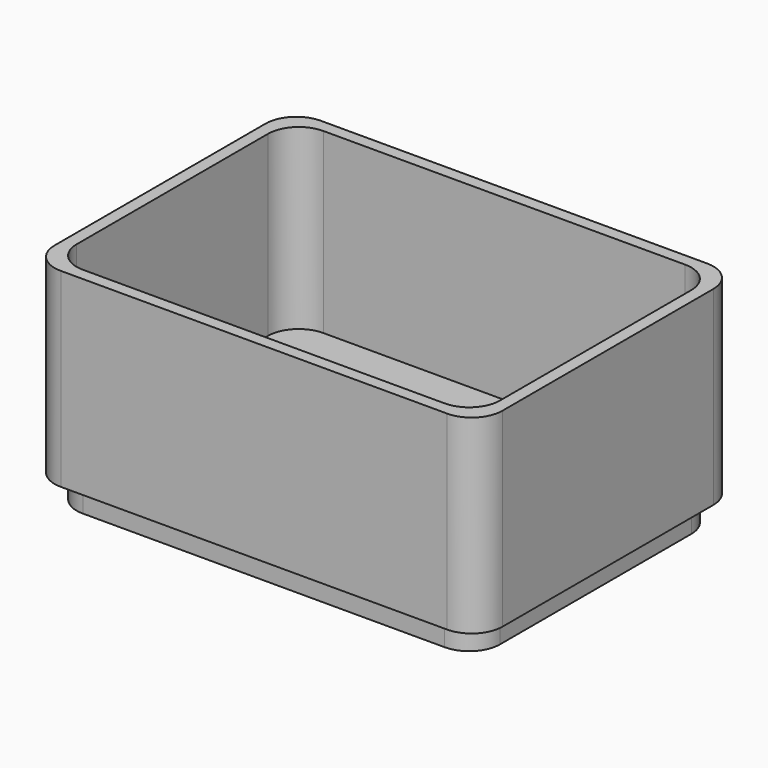
from build123d import *

# Parameters (mm, degrees)
F1_DEPTH = 6
F2_DEPTH = 35
F3_DEPTH = 4


with BuildPart() as f1:
    # F0 (on Top) → F1 (new body)
    with BuildSketch(Plane.XY):
        with BuildLine():
            Line((31.5, 26.5), (-31.5, 26.5))
            ThreePointArc((-31.5, 26.5), (-35.0355339059, 25.0355339059), (-36.5, 21.5))
            Line((-36.5, 21.5), (-36.5, -21.5))
            ThreePointArc((-36.5, -21.5), (-35.0355339059, -25.0355339059), (-31.5, -26.5))
            Line((-31.5, -26.5), (31.5, -26.5))
            ThreePointArc((31.5, -26.5), (35.0355339059, -25.0355339059), (36.5, -21.5))
            Line((36.5, -21.5), (36.5, 21.5))
            ThreePointArc((36.5, 21.5), (35.0355339059, 25.0355339059), (31.5, 26.5))
        make_face()
        with BuildLine():
            ThreePointArc((-34.5, 19.5), (-33.0355339059, 23.0355339059), (-29.5, 24.5))
            Line((-29.5, 24.5), (29.5, 24.5))
            ThreePointArc((29.5, 24.5), (33.0355339059, 23.0355339059), (34.5, 19.5))
            Line((34.5, 19.5), (34.5, -19.5))
            ThreePointArc((34.5, -19.5), (33.0355339059, -23.0355339059), (29.5, -24.5))
            Line((29.5, -24.5), (-29.5, -24.5))
            ThreePointArc((-29.5, -24.5), (-33.0355339059, -23.0355339059), (-34.5, -19.5))
            Line((-34.5, -19.5), (-34.5, 19.5))
        make_face(mode=Mode.SUBTRACT)
        with BuildLine():
            Line((29.5, 24.5), (-29.5, 24.5))
            ThreePointArc((-29.5, 24.5), (-33.0355339059, 23.0355339059), (-34.5, 19.5))
            Line((-34.5, 19.5), (-34.5, -19.5))
            ThreePointArc((-34.5, -19.5), (-33.0355339059, -23.0355339059), (-29.5, -24.5))
            Line((-29.5, -24.5), (29.5, -24.5))
            ThreePointArc((29.5, -24.5), (33.0355339059, -23.0355339059), (34.5, -19.5))
            Line((34.5, -19.5), (34.5, 19.5))
            ThreePointArc((34.5, 19.5), (33.0355339059, 23.0355339059), (29.5, 24.5))
        make_face()
    extrude(amount=F1_DEPTH)

    # F0 (on Top) → F2 (join)
    with BuildSketch(Plane.XY):
        with BuildLine():
            Line((31.5, 26.5), (-31.5, 26.5))
            ThreePointArc((-31.5, 26.5), (-35.0355339059, 25.0355339059), (-36.5, 21.5))
            Line((-36.5, 21.5), (-36.5, -21.5))
            ThreePointArc((-36.5, -21.5), (-35.0355339059, -25.0355339059), (-31.5, -26.5))
            Line((-31.5, -26.5), (31.5, -26.5))
            ThreePointArc((31.5, -26.5), (35.0355339059, -25.0355339059), (36.5, -21.5))
            Line((36.5, -21.5), (36.5, 21.5))
            ThreePointArc((36.5, 21.5), (35.0355339059, 25.0355339059), (31.5, 26.5))
        make_face()
        with BuildLine():
            ThreePointArc((-34.5, 19.5), (-33.0355339059, 23.0355339059), (-29.5, 24.5))
            Line((-29.5, 24.5), (29.5, 24.5))
            ThreePointArc((29.5, 24.5), (33.0355339059, 23.0355339059), (34.5, 19.5))
            Line((34.5, 19.5), (34.5, -19.5))
            ThreePointArc((34.5, -19.5), (33.0355339059, -23.0355339059), (29.5, -24.5))
            Line((29.5, -24.5), (-29.5, -24.5))
            ThreePointArc((-29.5, -24.5), (-33.0355339059, -23.0355339059), (-34.5, -19.5))
            Line((-34.5, -19.5), (-34.5, 19.5))
        make_face(mode=Mode.SUBTRACT)
    extrude(amount=F2_DEPTH)

    # F0 (on Top) → F3 (cut)
    with BuildSketch(Plane.XY):
        with BuildLine():
            Line((31.5, 26.5), (-31.5, 26.5))
            ThreePointArc((-31.5, 26.5), (-35.0355339059, 25.0355339059), (-36.5, 21.5))
            Line((-36.5, 21.5), (-36.5, -21.5))
            ThreePointArc((-36.5, -21.5), (-35.0355339059, -25.0355339059), (-31.5, -26.5))
            Line((-31.5, -26.5), (31.5, -26.5))
            ThreePointArc((31.5, -26.5), (35.0355339059, -25.0355339059), (36.5, -21.5))
            Line((36.5, -21.5), (36.5, 21.5))
            ThreePointArc((36.5, 21.5), (35.0355339059, 25.0355339059), (31.5, 26.5))
        make_face()
        with BuildLine():
            ThreePointArc((-34.5, 19.5), (-33.0355339059, 23.0355339059), (-29.5, 24.5))
            Line((-29.5, 24.5), (29.5, 24.5))
            ThreePointArc((29.5, 24.5), (33.0355339059, 23.0355339059), (34.5, 19.5))
            Line((34.5, 19.5), (34.5, -19.5))
            ThreePointArc((34.5, -19.5), (33.0355339059, -23.0355339059), (29.5, -24.5))
            Line((29.5, -24.5), (-29.5, -24.5))
            ThreePointArc((-29.5, -24.5), (-33.0355339059, -23.0355339059), (-34.5, -19.5))
            Line((-34.5, -19.5), (-34.5, 19.5))
        make_face(mode=Mode.SUBTRACT)
    extrude(amount=F3_DEPTH, mode=Mode.SUBTRACT)


solid = f1.part
